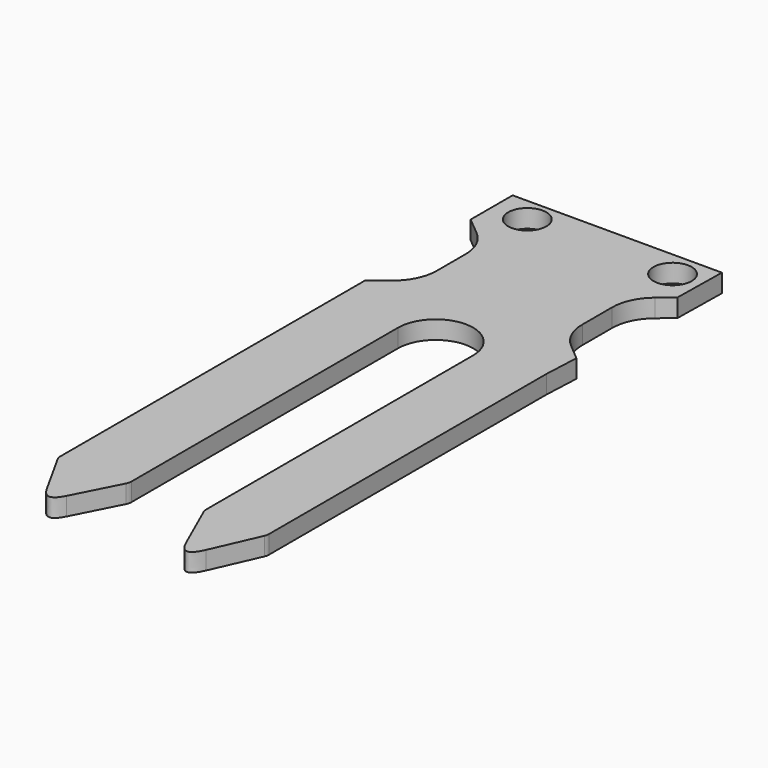
from build123d import *

# Parameters (mm, degrees)
F0_R         = 1.745
F1_DEPTH     = 1.66
F2_R         = 4
F3_T1_DEPTH  = 11.0406372139
F3_T3_DEPTH  = 2.9562992506
F3_T5_DEPTH  = 2.7192996153
F3_T7_DEPTH  = 12.9650408158
F3_T9_DEPTH  = 2.8625815694
F3_T11_DEPTH = 2.7133982533


# Not quite as in the source:
# - a fillet or chamfer that OpenCascade refuses, or shapes differently, is made with other operations: its cross-section is extruded or revolved along the edge and cut away or added


with BuildPart() as f1:
    # F0 (on Top) → F1 (new body)
    with BuildSketch(Plane.XY):
        with BuildLine():
            Line((9.301183783, 21.0652845629), (-9.82, 21.0652845629))
            Line((-9.82, 21.0652845629), (-9.82, 16.2710778286))
            Line((-9.82, 16.2710778286), (-6.76, 13.7425599752))
            Line((-6.76, 13.7425599752), (-6.76, 6.5925599752))
            Line((-6.76, 6.5925599752), (-9.82, 4.2610778286))
            Line((-9.82, 4.2610778286), (-9.82, 0.8810778286))
            Line((-9.82, 0.8810778286), (-9.82, -30.8189221714))
            Line((-9.82, -30.8189221714), (-6.5227223381, -36.7505173139))
            Line((-6.5227223381, -36.7505173139), (-3.43, -30.6931023543))
            Line((-3.43, -30.6931023543), (-3.43, 0))
            ThreePointArc((-3.43, 0), (0, 3.43), (3.43, 0))
            Line((3.43, 0), (3.43, -30.6931023543))
            Line((3.43, -30.6931023543), (6.4156440855, -37.4231023543))
            Line((6.4156440855, -37.4231023543), (9.301183783, -30.87889562))
            Line((9.301183783, -30.87889562), (9.301183783, 1.0068976457))
            Line((9.301183783, 1.0068976457), (9.4504277734, 4.2610778286))
            Line((9.4504277734, 4.2610778286), (6.5356440855, 6.7183797924))
            Line((6.5356440855, 6.7183797924), (6.5356440855, 13.8683797924))
            Line((6.5356440855, 13.8683797924), (9.2185314492, 16.0852845629))
            Line((9.2185314492, 16.0852845629), (9.301183783, 21.0652845629))
        make_face()
        with Locations((-6.686183783, 18.82610438)):
            Circle(F0_R, mode=Mode.SUBTRACT)
        with Locations((6.686183783, 18.7002845629)):
            Circle(F0_R, mode=Mode.SUBTRACT)
    extrude(amount=F1_DEPTH)

    # F2
    f2_edges = [f1.edges().sort_by_distance(p)[0] for p in [
        (-6.76, 6.59256, 0.83),
        (-6.76, 13.74256, 0.83),
        (6.535644, 6.71838, 0.83),
        (6.535644, 13.86838, 0.83),
    ]]
    fillet(f2_edges, radius=F2_R)

    # F3: fillet of radius 1 on 6 edges, made by hand

    # F3_s2 → F3_t1 (cut)
    with BuildSketch(Plane.XY.offset(-4.690318607)):
        with BuildLine():
            add(Edge.make_bspline(
                [(-7.4342616517, -35.110715417), (-6.5227223381, -36.7505173139), (-5.6695955837, -35.0795807734)],
                knots=[0, 0, 0, 1, 1, 1], degree=2, weights=[1, 1, 1]))
            Line((-5.6695955837, -35.0795807734), (-6.5227223381, -36.7505173139))
            Line((-6.5227223381, -36.7505173139), (-7.4342616517, -35.110715417))
        make_face()
    extrude(amount=F3_T1_DEPTH, mode=Mode.SUBTRACT)

    # F3_s4 → F3_t3 (cut)
    with BuildSketch(Plane.XY.offset(-0.6481496253)):
        with BuildLine():
            add(Edge.make_bspline(
                [(-9.82, -30.5596623213), (-9.82, -30.8189221714), (-9.6940354517, -31.0455244716)],
                knots=[0, 0, 0, 1, 1, 1], degree=2, weights=[1, 1, 1]))
            Line((-9.6940354517, -31.0455244716), (-9.82, -30.8189221714))
            Line((-9.82, -30.8189221714), (-9.82, -30.5596623213))
        make_face()
    extrude(amount=F3_T3_DEPTH, mode=Mode.SUBTRACT)

    # F3_s6 → F3_t5 (cut)
    with BuildSketch(Plane.XY.offset(-0.5296498077)):
        with BuildLine():
            add(Edge.make_bspline(
                [(3.43, -30.4812424312), (3.43, -30.6931023543), (3.5159130776, -30.8867607393)],
                knots=[0, 0, 0, 1, 1, 1], degree=2, weights=[1, 1, 1]))
            Line((3.5159130776, -30.8867607393), (3.43, -30.6931023543))
            Line((3.43, -30.6931023543), (3.43, -30.4812424312))
        make_face()
    extrude(amount=F3_T5_DEPTH, mode=Mode.SUBTRACT)

    # F3_s8 → F3_t7 (cut)
    with BuildSketch(Plane.XY.offset(-5.6525204079)):
        with BuildLine():
            add(Edge.make_bspline(
                [(5.4987638806, -35.3563443608), (6.4156440855, -37.4231023543), (7.3278517341, -35.3542777798)],
                knots=[0, 0, 0, 1, 1, 1], degree=2, weights=[1, 1, 1]))
            Line((7.3278517341, -35.3542777798), (6.4156440855, -37.4231023543))
            Line((6.4156440855, -37.4231023543), (5.4987638806, -35.3563443608))
        make_face()
    extrude(amount=F3_T7_DEPTH, mode=Mode.SUBTRACT)

    # F3_s10 → F3_t9 (cut)
    with BuildSketch(Plane.XY.offset(-0.6012907847)):
        with BuildLine():
            add(Edge.make_bspline(
                [(-3.5393693837, -30.9073135471), (-3.43, -30.6931023543), (-3.43, -30.4525860404)],
                knots=[0, 0, 0, 1, 1, 1], degree=2, weights=[1, 1, 1]))
            Line((-3.43, -30.4525860404), (-3.43, -30.6931023543))
            Line((-3.43, -30.6931023543), (-3.5393693837, -30.9073135471))
        make_face()
    extrude(amount=F3_T9_DEPTH, mode=Mode.SUBTRACT)

    # F3_s12 → F3_t11 (cut)
    with BuildSketch(Plane.XY.offset(-0.5266991266)):
        with BuildLine():
            add(Edge.make_bspline(
                [(9.301183783, -30.6682159693), (9.301183783, -30.87889562), (9.2161847141, -31.0716676965)],
                knots=[0, 0, 0, 1, 1, 1], degree=2, weights=[1, 1, 1]))
            Line((9.2161847141, -31.0716676965), (9.301183783, -30.87889562))
            Line((9.301183783, -30.87889562), (9.301183783, -30.6682159693))
        make_face()
    extrude(amount=F3_T11_DEPTH, mode=Mode.SUBTRACT)


solid = f1.part
